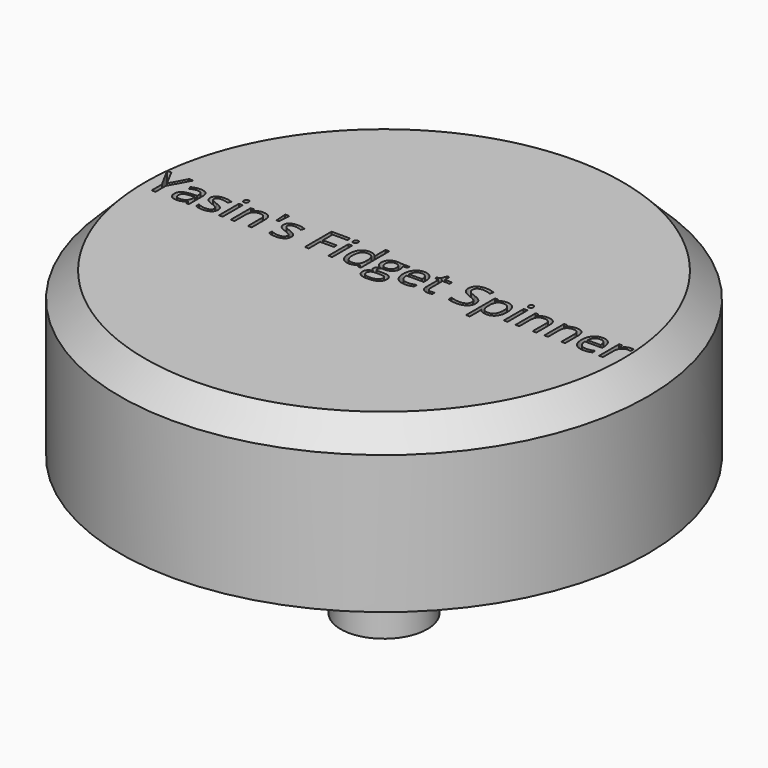
from build123d import *

# Parameters (mm, degrees)
F0_R         = 10.5
F1_DEPTH     = 4
F2_R         = 10
F3_DEPTH     = 2
F4_R         = 3.45
F4_R_2       = 1.725
F5_DEPTH     = 0.5
F6_DEPTH     = 7.5
F7_DEPTH     = 2.5
F8_SIZE      = 1
F9_TEXT_SIZE = 1.8596952048
F10_DEPTH    = 0.5


# Not quite as in the source:
# - Text() gives the source's letters only with a copy of the font that has no kerning and outlines rounded to 1/6400 em; it was checked with that copy


with BuildPart() as f1:
    # F0 (on Top) → F1 (new body)
    with BuildSketch(Plane.XY):
        Circle(F0_R)
    extrude(amount=F1_DEPTH)

    # F2 (on face) → F3 (cut)
    with BuildSketch(Plane(origin=(0, 0, 0), x_dir=(1, 0, 0), z_dir=(0, 0, -1))):
        Circle(F2_R)
    extrude(amount=-F3_DEPTH, mode=Mode.SUBTRACT)

    # F4 (on face) → F5 (join)
    with BuildSketch(Plane(origin=(0, 0, 2), x_dir=(1, 0, 0), z_dir=(0, 0, -1))):
        Circle(F4_R)
        Circle(F4_R_2, mode=Mode.SUBTRACT)
    extrude(amount=F5_DEPTH)

    # F6 (add): a face of the model
    f6_faces = [f1.faces().sort_by_distance(p)[0] for p in [
        (0, 0, 2),
    ]]
    extrude(f6_faces, amount=F6_DEPTH)

    # F7 (add): a face of the model
    f7_faces = [f1.faces().sort_by_distance(p)[0] for p in [
        (0, 0, 4),
    ]]
    extrude(f7_faces, amount=F7_DEPTH)

    # F8
    f8_edges = [f1.edges().sort_by_distance(p)[0] for p in [
        (-10.5, 0, 6.5),
    ]]
    chamfer(f8_edges, length=F8_SIZE)

    # F9 (on face) → F10 (cut)
    with BuildSketch(Plane.XY.offset(6.5)):
        with Locations((-9.4435705347, -0.3050678066)):
            Text("Yasin's Fidget Spinner", F9_TEXT_SIZE, font='Open Sans', text_align=(TextAlign.LEFT, TextAlign.BOTTOM))
    extrude(amount=-F10_DEPTH, mode=Mode.SUBTRACT)


solid = f1.part
